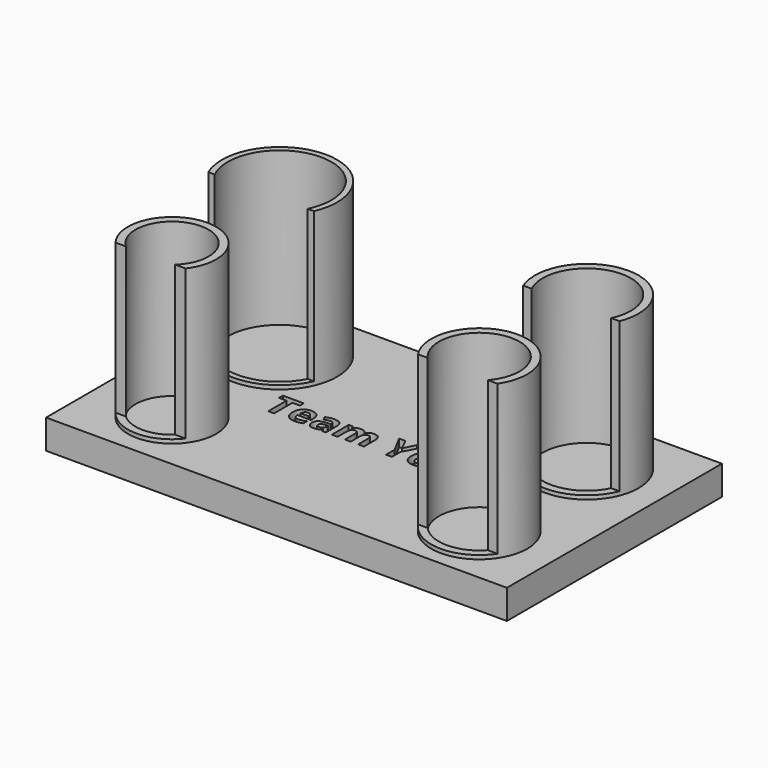
from build123d import *

# Parameters (mm, degrees)
F0_W          = 120
F0_H          = 70
F1_DEPTH      = 7.62
F2_R          = 15
F2_R_2        = 13.5
F3_DEPTH      = 40
F2_R_3        = 11.5
F4_DEPTH      = 40
F2_R_4        = 12.5
F2_R_5        = 10.5
F5_DEPTH      = 40
F2_R_6        = 9.5
F6_DEPTH      = 40
F8_DEPTH      = 39
F10_DEPTH     = 39
F12_DEPTH     = 39
F14_DEPTH     = 39
F15_TEXT_SIZE = 10.0962296892
F16_DEPTH     = 2
F17_DEPTH     = 39
F18_DEPTH     = 39
F19_DEPTH     = 39
F20_DEPTH     = 39


# Not quite as in the source:
# - Text() gives the source's letters only with a copy of the font that has no kerning and outlines rounded to 1/6400 em; it was checked with that copy


with BuildPart() as f1:
    # F0 (on Top) → F1 (new body)
    with BuildSketch(Plane.XY):
        Rectangle(F0_W, F0_H)
    extrude(amount=F1_DEPTH)

    # F2 (on face) → F3 (join)
    with BuildSketch(Plane.XY.offset(7.62)):
        with Locations((-40, 16)):
            Circle(F2_R)
        with Locations((-40, 16)):
            Circle(F2_R_2, mode=Mode.SUBTRACT)
    extrude(amount=F3_DEPTH)

    # F2 (on face) → F4 (join)
    with BuildSketch(Plane.XY.offset(7.62)):
        with Locations((40, 16)):
            Circle(F2_R_2)
        with Locations((40, 16)):
            Circle(F2_R_3, mode=Mode.SUBTRACT)
    extrude(amount=F4_DEPTH)

    # F2 (on face) → F5 (join)
    with BuildSketch(Plane.XY.offset(7.62)):
        with Locations((40, -19)):
            Circle(F2_R_4)
        with Locations((40, -19)):
            Circle(F2_R_5, mode=Mode.SUBTRACT)
    extrude(amount=F5_DEPTH)

    # F2 (on face) → F6 (join)
    with BuildSketch(Plane.XY.offset(7.62)):
        with Locations((-40, -19)):
            Circle(F2_R_3)
        with Locations((-40, -19)):
            Circle(F2_R_6, mode=Mode.SUBTRACT)
    extrude(amount=F6_DEPTH)

    # F7 (on face) → F8 (cut)
    with BuildSketch(Plane.XY.offset(47.62)):
        with BuildLine():
            Line((-52.0933866224, 10), (-53.7477270849, 10))
            ThreePointArc((-53.7477270849, 10), (-40, 1), (-26.2522729151, 10))
            Line((-26.2522729151, 10), (-27.9066133776, 10))
            ThreePointArc((-27.9066133776, 10), (-40, 2.5), (-52.0933866224, 10))
        make_face()
    extrude(amount=-F8_DEPTH, mode=Mode.SUBTRACT)

    # F9 (on face) → F10 (cut)
    with BuildSketch(Plane.XY.offset(47.62)):
        with BuildLine():
            Line((29.6438424114, 11), (27.460063796, 11))
            ThreePointArc((27.460063796, 11), (30.0048706296, 6.9254537926), (33.8153415616, 4))
            Line((33.8153415616, 4), (46.1846584384, 4))
            ThreePointArc((46.1846584384, 4), (49.9951293704, 6.9254537926), (52.539936204, 11))
            Line((52.539936204, 11), (50.3561575886, 11))
            ThreePointArc((50.3561575886, 11), (40, 4.5), (29.6438424114, 11))
        make_face()
    extrude(amount=-F10_DEPTH, mode=Mode.SUBTRACT)

    # F11 (on face) → F12 (cut)
    with BuildSketch(Plane.XY.offset(47.62)):
        with BuildLine():
            Line((-46.4226162893, -26), (-49.1241437954, -26))
            ThreePointArc((-49.1241437954, -26), (-46.5518435819, -28.4511028816), (-43.3541019663, -30))
            Line((-43.3541019663, -30), (-36.6458980338, -30))
            ThreePointArc((-36.6458980338, -30), (-33.4481564181, -28.4511028816), (-30.8758562046, -26))
            Line((-30.8758562046, -26), (-33.5773837107, -26))
            ThreePointArc((-33.5773837107, -26), (-40, -28.5), (-46.4226162893, -26))
        make_face()
    extrude(amount=-F12_DEPTH, mode=Mode.SUBTRACT)

    # F13 (on face) → F14 (cut)
    with BuildSketch(Plane.XY.offset(47.62)):
        with BuildLine():
            Line((32.1737620788, -26), (29.6438424114, -26))
            ThreePointArc((29.6438424114, -26), (40, -31.5), (50.3561575886, -26))
            Line((50.3561575886, -26), (47.8262379212, -26))
            ThreePointArc((47.8262379212, -26), (40, -29.5), (32.1737620788, -26))
        make_face()
    extrude(amount=-F14_DEPTH, mode=Mode.SUBTRACT)

    # F15 (on face) → F16 (cut)
    with BuildSketch(Plane.XY.offset(7.62)):
        with Locations((-28.629699544, -4.5780207272)):
            Text('Team Yeezy', F15_TEXT_SIZE, font='Open Sans', font_style=FontStyle.BOLD, text_align=(TextAlign.LEFT, TextAlign.BOTTOM))
    extrude(amount=-F16_DEPTH, mode=Mode.SUBTRACT)

    # F17 (add): a face of the model
    f17_faces = [f1.faces().sort_by_distance(p)[0] for p in [
        (40, 3.3970478561, 47.62),
    ]]
    extrude(f17_faces, amount=F17_DEPTH)

    # F18 (cut): a face of the model
    f18_faces = [f1.faces().sort_by_distance(p)[0] for p in [
        (-40, -30.2003774159, 47.62),
    ]]
    extrude(f18_faces, amount=-F18_DEPTH, mode=Mode.SUBTRACT)

    # F19 (cut): a face of the model
    f19_faces = [f1.faces().sort_by_distance(p)[0] for p in [
        (40, 3.3970478561, 86.62),
    ]]
    extrude(f19_faces, amount=-F19_DEPTH, mode=Mode.SUBTRACT)

    # F20 (cut): a face of the model
    f20_faces = [f1.faces().sort_by_distance(p)[0] for p in [
        (40, 3.3970478561, 47.62),
    ]]
    extrude(f20_faces, amount=-F20_DEPTH, mode=Mode.SUBTRACT)


solid = f1.part
